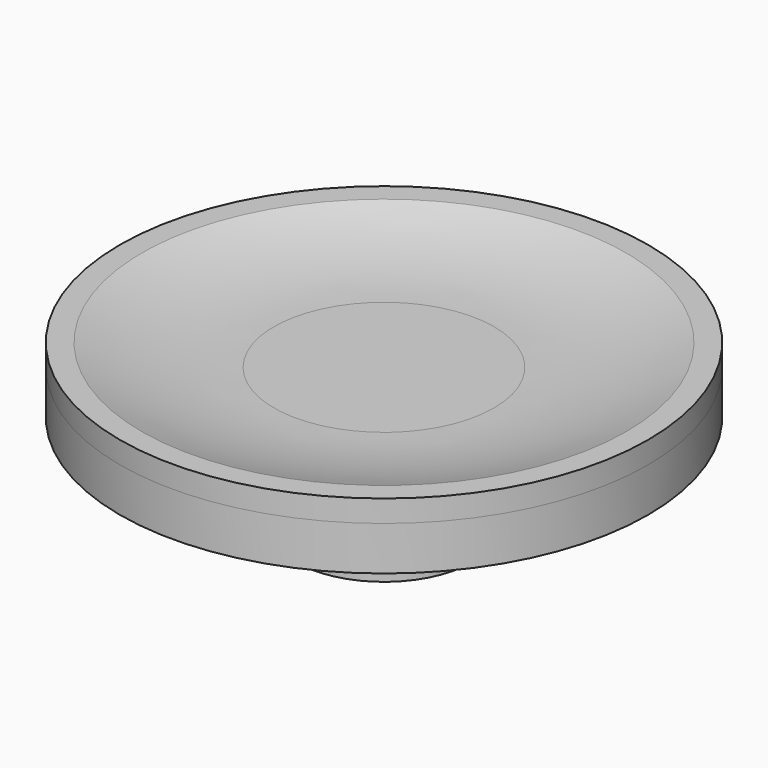
from build123d import *


# Not quite as in the source:
# - a feature of the source that left no trace in its solid (it failed there, or was rolled back) is left out
# - a feature names something its author has since deleted; it is built from what else it names


with BuildPart() as f1:
    # F0 (on Front) → F1 (revolve)
    with BuildSketch(Plane.XZ):
        Polygon((0, 5.5), (0, 0), (4, 0), (4, 3.5), (5, 4.5), (12, 4.5), (12, 6.5), (11, 5.5), align=None)
    revolve(axis=Axis((0, 0, 2.75), (0, 0, -1)))


with BuildPart() as f2:
    # F0 (on Front) → F2 (revolve)
    with BuildSketch(Plane.XZ):
        with BuildLine():
            Line((0, 6.5), (0, 5.5))
            Line((0, 5.5), (11, 5.5))
            Line((11, 5.5), (12, 6.5))
            Line((12, 6.5), (12, 7.5))
            Line((12, 7.5), (11, 7.5))
            ThreePointArc((11, 7.5), (8.0413812651, 6.7517124091), (5, 6.5))
            Line((5, 6.5), (0, 6.5))
        make_face()
    revolve(axis=Axis((0, 0, 2.75), (0, 0, -1)))


solid = Compound([f1.part, f2.part])
